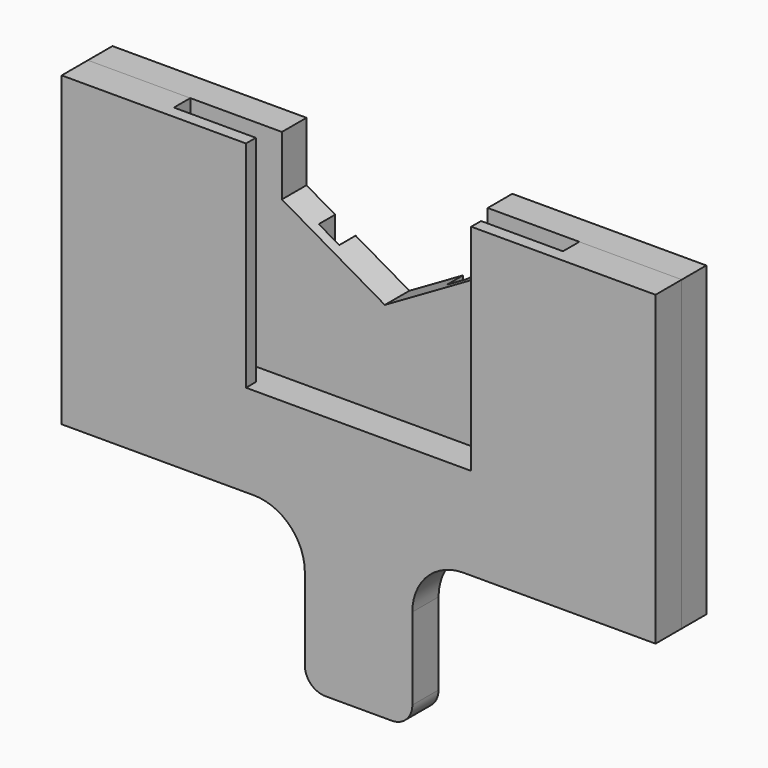
from build123d import *

# Parameters (mm, degrees)
F0_W      = 38
F0_H      = 1.2
F1_DEPTH  = 20
F3_W      = 10
F3_H      = 20
F4_DEPTH  = 3.2
F5_W      = 10
F5_H      = 20
F6_DEPTH  = 3.2
F7_W      = 38
F7_H      = 2
F8_DEPTH  = 10
F2_W      = 22
F2_H      = 1.2
F9_DEPTH  = 20
F10_W     = 3
F10_H     = 30
F11_DEPTH = 58
F13_DEPTH = 6.201
F15_DEPTH = 2
F16_W     = 10.5
F16_H     = 3.2
F17_DEPTH = 15
F18_R     = 5
F19_R     = 2
F20_DEPTH = 1


with BuildPart() as f1:
    # F0 (on Top) → F1 (new body)
    with BuildSketch(Plane.XY):
        with Locations((19, 0.6)):
            Rectangle(F0_W, F0_H)
    extrude(amount=F1_DEPTH)

    # F3 (on face) → F4 (join)
    with BuildSketch(Plane.XZ):
        with Locations((-5, 10)):
            Rectangle(F3_W, F3_H)
    extrude(amount=-F4_DEPTH)

    # F5 (on face) → F6 (join)
    with BuildSketch(Plane.XZ):
        with Locations((43, 10)):
            Rectangle(F5_W, F5_H)
    extrude(amount=-F6_DEPTH)

    # F7 (on face) → F8 (join)
    with BuildSketch(Plane(origin=(0, 0, 0), x_dir=(1, 0, 0), z_dir=(0, 0, -1))):
        with Locations((19, -2.2)):
            Rectangle(F7_W, F7_H)
        Polygon((48, -3.2), (48, 0), (-10, 0), (-10, -3.2), (0, -3.2), (0, -1.2), (38, -1.2), (38, -3.2), align=None)
    extrude(amount=F8_DEPTH)

    # F2 (on face) → F9 (cut)
    with BuildSketch(Plane.XY.offset(20)):
        with Locations((19, 0.6)):
            Rectangle(F2_W, F2_H)
    extrude(amount=-F9_DEPTH, mode=Mode.SUBTRACT)

    # F16 (on face) → F17 (join)
    with BuildSketch(Plane(origin=(0, 0, -10), x_dir=(1, 0, 0), z_dir=(0, 0, -1))):
        with Locations((19, -1.6)):
            Rectangle(F16_W, F16_H)
    extrude(amount=F17_DEPTH)

    # F18
    f18_edges = [f1.edges().sort_by_distance(p)[0] for p in [
        (24.25, 1.6, -10),
        (13.75, 1.6, -10),
    ]]
    fillet(f18_edges, radius=F18_R)

    # F19
    f19_edges = [f1.edges().sort_by_distance(p)[0] for p in [
        (24.25, 1.6, -25),
        (13.75, 1.6, -25),
    ]]
    fillet(f19_edges, radius=F19_R)

    # F20 (cut): a face of the model
    f20_faces = [f1.faces().sort_by_distance(p)[0] for p in [
        (19, 1.7875, 0),
    ]]
    extrude(f20_faces, amount=-F20_DEPTH, mode=Mode.SUBTRACT)


with BuildPart() as f11:
    # F10 (on face) → F11 (new body)
    with BuildSketch(Plane.YZ.offset(48)):
        with Locations((4.7, 5)):
            Rectangle(F10_W, F10_H)
    extrude(amount=-F11_DEPTH)

    # F12 (on face) → F13 (cut, through all)
    with BuildSketch(Plane(origin=(0, 6.2, 0), x_dir=(-1, 0, 0), z_dir=(0, 1, 0))):
        Polygon((-29.05, 20), (-29.05, 14.1976297946), (-19, 8.3952595893), (-8.95, 14.1976297946), (-8.95, 20), align=None)
    extrude(amount=-F13_DEPTH, mode=Mode.SUBTRACT)

    # F14 (on face) → F15 (cut)
    with BuildSketch(Plane(origin=(0, 6.2, 0), x_dir=(-1, 0, 0), z_dir=(0, 1, 0))):
        Polygon((-24.25, 11.1954083949), (-26.25, 12.3501089332), (-26.25, -16.1530785263), (-24.25, -16.2737797946), align=None)
        Polygon((-26.25, 13.1725249812), (-26.25, 12.3501089332), (-24.25, 11.1954083949), (-24.25, 13.1725249812), align=None)
        Polygon((-11.75, -16.6962388903), (-11.75, 12.3501089332), (-11.75, 12.5810490409), (-13.75, 12.8753753379), (-13.75, 11.1954083949), (-13.75, -16.0927250981), align=None)
    extrude(amount=-F15_DEPTH, mode=Mode.SUBTRACT)


solid = Compound([f1.part, f11.part])
